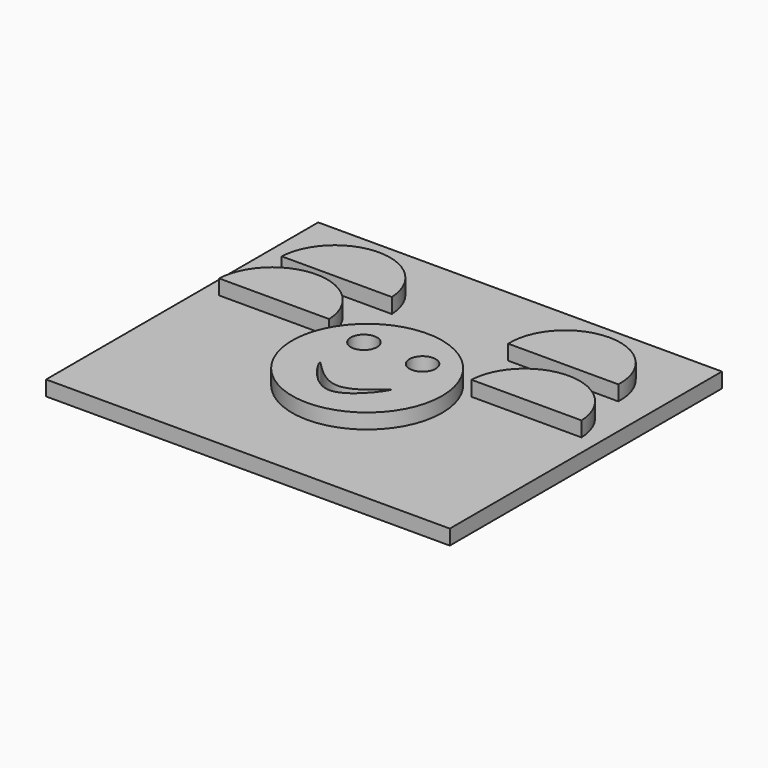
from build123d import *

# Parameters (mm, degrees)
F0_W     = 136.8003189564
F0_H     = 115.2591593564
F0_R     = 25.413882958
F1_DEPTH = 5.08
F2_DEPTH = 10.16
F0_R_2   = 4.445
F3_DEPTH = 10.16


# Not quite as in the source:
# - the program builds the solid bodies; features that only make, move or delete a surface that nothing else refers to are left out


with BuildPart() as f1:
    # F0 (on Top) → F1 (new body)
    with BuildSketch(Plane.XY):
        with Locations((0, 7.1337576956)):
            Rectangle(F0_W, F0_H)
        Circle(F0_R, mode=Mode.SUBTRACT)
        with BuildLine():
            Line((-25.4373313075, 15.699069947), (-62.7512871141, 15.699069947))
            ThreePointArc((-62.7512871141, 15.699069947), (-44.0943092108, 33.5629857305), (-25.4373313075, 15.699069947))
        make_face(mode=Mode.SUBTRACT)
        with BuildLine():
            Line((-20.3688811746, 35.9205551982), (-57.6828369811, 35.9205551982))
            ThreePointArc((-57.6828369811, 35.9205551982), (-39.0258590779, 53.7844709817), (-20.3688811746, 35.9205551982))
        make_face(mode=Mode.SUBTRACT)
        with BuildLine():
            Line((62.9981844539, 12.06225143), (25.6842286473, 12.06225143))
            ThreePointArc((25.6842286473, 12.06225143), (44.3412065506, 29.9261672135), (62.9981844539, 12.06225143))
        make_face(mode=Mode.SUBTRACT)
        with BuildLine():
            ThreePointArc((20.3699840242, 34.2742279379), (39.0258590779, 53.7844709817), (57.6817341315, 34.2742279379))
            Line((57.6817341315, 34.2742279379), (20.3699840242, 34.2742279379))
        make_face(mode=Mode.SUBTRACT)
    extrude(amount=F1_DEPTH)

    # F0 (on Top) → F2 (join)
    with BuildSketch(Plane.XY):
        with BuildLine():
            ThreePointArc((-20.3688811746, 35.9205551982), (-39.0258590779, 53.7844709817), (-57.6828369811, 35.9205551982))
            Line((-57.6828369811, 35.9205551982), (-20.3688811746, 35.9205551982))
        make_face()
        with BuildLine():
            ThreePointArc((-25.4373313075, 15.699069947), (-44.0943092108, 33.5629857305), (-62.7512871141, 15.699069947))
            Line((-62.7512871141, 15.699069947), (-25.4373313075, 15.699069947))
        make_face()
        with BuildLine():
            Line((20.3699840242, 34.2742279379), (57.6817341315, 34.2742279379))
            ThreePointArc((57.6817341315, 34.2742279379), (39.0258590779, 53.7844709817), (20.3699840242, 34.2742279379))
        make_face()
        with BuildLine():
            ThreePointArc((62.9981844539, 12.06225143), (44.3412065506, 29.9261672135), (25.6842286473, 12.06225143))
            Line((25.6842286473, 12.06225143), (62.9981844539, 12.06225143))
        make_face()
    extrude(amount=F2_DEPTH)

    # F0 (on Top) → F3 (join)
    with BuildSketch(Plane.XY):
        Circle(F0_R)
        with BuildLine():
            add(Edge.make_bspline(
                [(-11.889597401, -5.1754722372), (-11.6308932935, -4.6629733601), (-0.1804625636, -20.6748608417), (19.2699362073, 3.5560661133), (-0.2450377996, -26.2958289114), (-12.1664951894, -5.7240132208), (-11.889597401, -5.1754722372)],
                knots=[0, 0, 0, 0, 0.2394881843, 0.4838109378, 0.743669518, 1, 1, 1, 1], degree=3))
        make_face(mode=Mode.SUBTRACT)
        with Locations((-9.9313119426, 11.0503323376)):
            Circle(F0_R_2, mode=Mode.SUBTRACT)
        with Locations((9.9313119426, 11.0503323376)):
            Circle(F0_R_2, mode=Mode.SUBTRACT)
    extrude(amount=F3_DEPTH)


solid = f1.part
